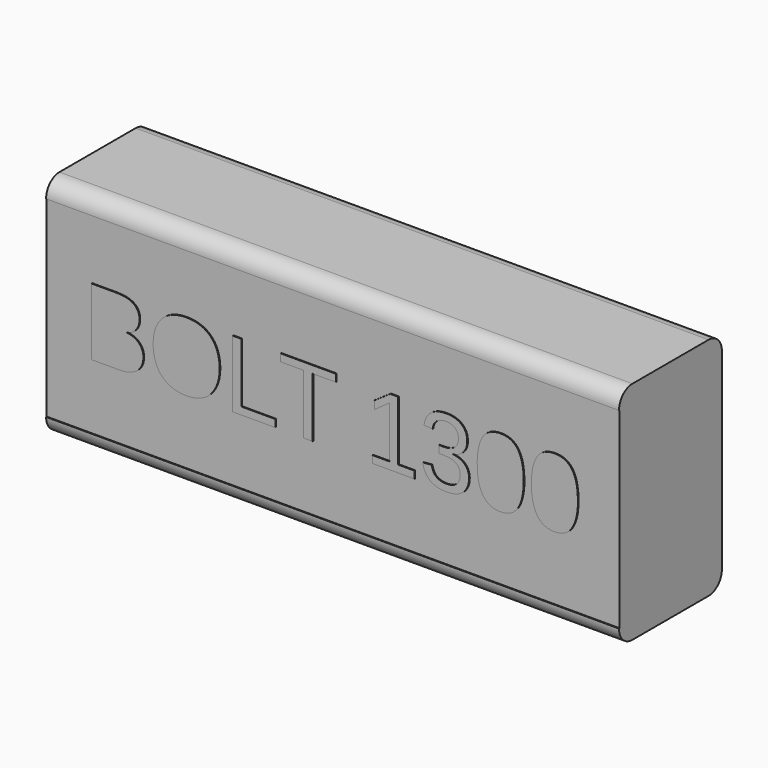
from build123d import *

# Parameters (mm, degrees)
F0_W     = 87.122
F0_H     = 34.29
F1_DEPTH = 9.779
F2_R     = 2.54
F3_W     = 87.122
F3_H     = 29.21
F4_DEPTH = 0.127


with BuildPart() as f1:
    # F0 (on Front) → F1 (new body, symmetric)
    with BuildSketch(Plane.XZ):
        Rectangle(F0_W, F0_H)
    extrude(amount=F1_DEPTH, both=True)

    # F2
    f2_edges = [f1.edges().sort_by_distance(p)[0] for p in [
        (0, 9.779, 17.145),
        (0, 9.779, -17.145),
        (0, -9.779, 17.145),
        (0, -9.779, -17.145),
    ]]
    fillet(f2_edges, radius=F2_R)

    # F3 (on face) → F4 (cut)
    with BuildSketch(Plane.XZ.offset(9.779)):
        Rectangle(F3_W, F3_H)
        with BuildLine():
            add(Edge.make_bspline(
                [(-29.4201796663, -0.1257045448), (-28.7628641118, -0.7945925563), (-28.7628641118, -1.8129687674)],
                knots=[0, 0, 0, 1, 1, 1], degree=2))
            add(Edge.make_bspline(
                [(-28.7628641118, -1.8129687674), (-28.7628641118, -3.1738897042), (-29.7534664263, -3.9295711427)],
                knots=[0, 0, 0, 1, 1, 1], degree=2))
            add(Edge.make_bspline(
                [(-29.7534664263, -3.9295711427), (-30.7440687408, -4.6852525812), (-32.5077111792, -4.6852525812)],
                knots=[0, 0, 0, 1, 1, 1], degree=2))
            Line((-32.5077111792, -4.6852525812), (-36.6460217827, -4.6852525812))
            Line((-36.6460217827, -4.6852525812), (-36.6460217827, 5.5054530046))
            Line((-36.6460217827, 5.5054530046), (-32.9428355603, 5.5054530046))
            add(Edge.make_bspline(
                [(-32.9428355603, 5.5054530046), (-29.3553739074, 5.5054530046), (-29.3553739074, 3.0312617097)],
                knots=[0, 0, 0, 1, 1, 1], degree=2))
            add(Edge.make_bspline(
                [(-29.3553739074, 3.0312617097), (-29.3553739074, 2.128610068), (-29.8610902759, 1.5141126043)],
                knots=[0, 0, 0, 1, 1, 1], degree=2))
            add(Edge.make_bspline(
                [(-29.8610902759, 1.5141126043), (-30.3668066444, 0.8996151405), (-31.2926032, 0.6889964241)],
                knots=[0, 0, 0, 1, 1, 1], degree=2))
            add(Edge.make_bspline(
                [(-31.2926032, 0.6889964241), (-30.0774952208, 0.5431834666), (-29.4201796663, -0.1257045448)],
                knots=[0, 0, 0, 1, 1, 1], degree=2))
        make_face(mode=Mode.SUBTRACT)
        with BuildLine():
            add(Edge.make_bspline(
                [(-17.7713445055, 3.2418804261), (-17.1672622529, 2.0638043091), (-17.1672622529, 0.4575472852)],
                knots=[0, 0, 0, 1, 1, 1], degree=2))
            add(Edge.make_bspline(
                [(-17.1672622529, 0.4575472852), (-17.1672622529, -1.1417662646), (-17.7782879796, -2.3418300498)],
                knots=[0, 0, 0, 1, 1, 1], degree=2))
            add(Edge.make_bspline(
                [(-17.7782879796, -2.3418300498), (-18.3893137063, -3.541893835), (-19.5326724525, -4.1864796868)],
                knots=[0, 0, 0, 1, 1, 1], degree=2))
            add(Edge.make_bspline(
                [(-19.5326724525, -4.1864796868), (-20.6760311986, -4.8310655387), (-22.2313694121, -4.8310655387)],
                knots=[0, 0, 0, 1, 1, 1], degree=2))
            add(Edge.make_bspline(
                [(-22.2313694121, -4.8310655387), (-23.8005945738, -4.8310655387), (-24.9393243372, -4.193423161)],
                knots=[0, 0, 0, 1, 1, 1], degree=2))
            add(Edge.make_bspline(
                [(-24.9393243372, -4.193423161), (-26.0780541006, -3.5557807833), (-26.678664616, -2.3522452611)],
                knots=[0, 0, 0, 1, 1, 1], degree=2))
            add(Edge.make_bspline(
                [(-26.678664616, -2.3522452611), (-27.2792751315, -1.1487097388), (-27.2792751315, 0.4575472852)],
                knots=[0, 0, 0, 1, 1, 1], degree=2))
            add(Edge.make_bspline(
                [(-27.2792751315, 0.4575472852), (-27.2792751315, 2.901650192), (-25.9414991086, 4.2799298141)],
                knots=[0, 0, 0, 1, 1, 1], degree=2))
            add(Edge.make_bspline(
                [(-25.9414991086, 4.2799298141), (-24.6037230858, 5.6582094363), (-22.2151679723, 5.6582094363)],
                knots=[0, 0, 0, 1, 1, 1], degree=2))
            add(Edge.make_bspline(
                [(-22.2151679723, 5.6582094363), (-20.6598297589, 5.6582094363), (-19.5176282585, 5.0390829897)],
                knots=[0, 0, 0, 1, 1, 1], degree=2))
            add(Edge.make_bspline(
                [(-19.5176282585, 5.0390829897), (-18.375426758, 4.4199565431), (-17.7713445055, 3.2418804261)],
                knots=[0, 0, 0, 1, 1, 1], degree=2))
        make_face(mode=Mode.SUBTRACT)
        Polygon((-8.7124252089, -4.6852525812), (-15.2439199087, -4.6852525812), (-15.2439199087, 5.5054530046), (-13.8621685494, 5.5054530046), (-13.8621685494, -3.5557807833), (-8.7124252089, -3.5557807833), align=None, mode=Mode.SUBTRACT)
        Polygon((0.4876780624, 4.3782956981), (-3.0141474092, 4.3782956981), (-3.0141474092, -4.6852525812), (-4.3889552943, -4.6852525812), (-4.3889552943, 4.3782956981), (-7.8884662744, 4.3782956981), (-7.8884662744, 5.5054530046), (0.4876780624, 5.5054530046), align=None, mode=Mode.SUBTRACT)
        Polygon((12.4559130349, -4.6852525812), (6.0702312926, -4.6852525812), (6.0702312926, -3.5789256972), (8.6647761397, -3.5789256972), (8.6647761397, 4.2625711287), (6.3664861904, 2.6192822425), (6.3664861904, 3.8505916615), (8.773557235, 5.5054530046), (9.9747782659, 5.5054530046), (9.9747782659, -3.5789256972), (12.4559130349, -3.5789256972), align=None, mode=Mode.SUBTRACT)
        with BuildLine():
            add(Edge.make_bspline(
                [(20.1284519894, -0.2506870799), (20.7649371214, -0.894115686), (20.7649371214, -1.8708310521)],
                knots=[0, 0, 0, 1, 1, 1], degree=2))
            add(Edge.make_bspline(
                [(20.7649371214, -1.8708310521), (20.7649371214, -3.2826707994), (19.8680717081, -4.0568681691)],
                knots=[0, 0, 0, 1, 1, 1], degree=2))
            add(Edge.make_bspline(
                [(19.8680717081, -4.0568681691), (18.9712062949, -4.8310655387), (17.3070869862, -4.8310655387)],
                knots=[0, 0, 0, 1, 1, 1], degree=2))
            add(Edge.make_bspline(
                [(17.3070869862, -4.8310655387), (15.7610067384, -4.8310655387), (14.8386819198, -4.1320891392)],
                knots=[0, 0, 0, 1, 1, 1], degree=2))
            add(Edge.make_bspline(
                [(14.8386819198, -4.1320891392), (13.9163571013, -3.4331127397), (13.7427702471, -2.0675628202)],
                knots=[0, 0, 0, 1, 1, 1], degree=2))
            Line((13.7427702471, -2.0675628202), (15.0874897442, -1.9448947766))
            add(Edge.make_bspline(
                [(15.0874897442, -1.9448947766), (15.3490272711, -3.7525125514), (17.3070869862, -3.7525125514)],
                knots=[0, 0, 0, 1, 1, 1], degree=2))
            add(Edge.make_bspline(
                [(17.3070869862, -3.7525125514), (18.2907458265, -3.7525125514), (18.8520099884, -3.2676266054)],
                knots=[0, 0, 0, 1, 1, 1], degree=2))
            add(Edge.make_bspline(
                [(18.8520099884, -3.2676266054), (19.4132741502, -2.7827406594), (19.4132741502, -1.8291702071)],
                knots=[0, 0, 0, 1, 1, 1], degree=2))
            add(Edge.make_bspline(
                [(19.4132741502, -1.8291702071), (19.4132741502, -0.9959533071), (18.7733172811, -0.5295832922)],
                knots=[0, 0, 0, 1, 1, 1], degree=2))
            add(Edge.make_bspline(
                [(18.7733172811, -0.5295832922), (18.1333604121, -0.0632132773), (16.925195907, -0.0632132773)],
                knots=[0, 0, 0, 1, 1, 1], degree=2))
            Line((16.925195907, -0.0632132773), (16.1868731539, -0.0632132773))
            Line((16.1868731539, -0.0632132773), (16.1868731539, 1.0639440291))
            Line((16.1868731539, 1.0639440291), (16.895107519, 1.0639440291))
            add(Edge.make_bspline(
                [(16.895107519, 1.0639440291), (17.9667170321, 1.0639440291), (18.5557550906, 1.5314712897)],
                knots=[0, 0, 0, 1, 1, 1], degree=2))
            add(Edge.make_bspline(
                [(18.5557550906, 1.5314712897), (19.1447931491, 1.9989985503), (19.1447931491, 2.8229574847)],
                knots=[0, 0, 0, 1, 1, 1], degree=2))
            add(Edge.make_bspline(
                [(19.1447931491, 2.8229574847), (19.1447931491, 3.6399729451), (18.6645361859, 4.1132864341)],
                knots=[0, 0, 0, 1, 1, 1], degree=2))
            add(Edge.make_bspline(
                [(18.6645361859, 4.1132864341), (18.1842792226, 4.5865999232), (17.2353377531, 4.5865999232)],
                knots=[0, 0, 0, 1, 1, 1], degree=2))
            add(Edge.make_bspline(
                [(17.2353377531, 4.5865999232), (16.3743469564, 4.5865999232), (15.8431711827, 4.1456893136)],
                knots=[0, 0, 0, 1, 1, 1], degree=2))
            add(Edge.make_bspline(
                [(15.8431711827, 4.1456893136), (15.3119954089, 3.7047787039), (15.2240447361, 2.901650192)],
                knots=[0, 0, 0, 1, 1, 1], degree=2))
            Line((15.2240447361, 2.901650192), (13.9163571013, 3.0034878131))
            add(Edge.make_bspline(
                [(13.9163571013, 3.0034878131), (14.0598555674, 4.2556276545), (14.9532492436, 4.9569185454)],
                knots=[0, 0, 0, 1, 1, 1], degree=2))
            add(Edge.make_bspline(
                [(14.9532492436, 4.9569185454), (15.8466429197, 5.6582094363), (17.2492247015, 5.6582094363)],
                knots=[0, 0, 0, 1, 1, 1], degree=2))
            add(Edge.make_bspline(
                [(17.2492247015, 5.6582094363), (18.7837324924, 5.6582094363), (19.6331508322, 4.9453460885)],
                knots=[0, 0, 0, 1, 1, 1], degree=2))
            add(Edge.make_bspline(
                [(19.6331508322, 4.9453460885), (20.4825691719, 4.2324827406), (20.4825691719, 2.9595124767)],
                knots=[0, 0, 0, 1, 1, 1], degree=2))
            add(Edge.make_bspline(
                [(20.4825691719, 2.9595124767), (20.4825691719, 1.9827971105), (19.9363492041, 1.3717713838)],
                knots=[0, 0, 0, 1, 1, 1], degree=2))
            add(Edge.make_bspline(
                [(19.9363492041, 1.3717713838), (19.3901292363, 0.7607456571), (18.3486081113, 0.5431834666)],
                knots=[0, 0, 0, 1, 1, 1], degree=2))
            Line((18.3486081113, 0.5431834666), (18.3486081113, 0.5154095699))
            add(Edge.make_bspline(
                [(18.3486081113, 0.5154095699), (19.4919668574, 0.3927415263), (20.1284519894, -0.2506870799)],
                knots=[0, 0, 0, 1, 1, 1], degree=2))
        make_face(mode=Mode.SUBTRACT)
        with BuildLine():
            add(Edge.make_bspline(
                [(28.2175993939, 4.3343203618), (29.0739612079, 3.0104312872), (29.0739612079, 0.4135719488)],
                knots=[0, 0, 0, 1, 1, 1], degree=2))
            add(Edge.make_bspline(
                [(29.0739612079, 0.4135719488), (29.0739612079, -2.1393120533), (28.1736240576, -3.485188796)],
                knots=[0, 0, 0, 1, 1, 1], degree=2))
            add(Edge.make_bspline(
                [(28.1736240576, -3.485188796), (27.2732869072, -4.8310655387), (25.516587943, -4.8310655387)],
                knots=[0, 0, 0, 1, 1, 1], degree=2))
            add(Edge.make_bspline(
                [(25.516587943, -4.8310655387), (23.7598889787, -4.8310655387), (22.8769105138, -3.4921322701)],
                knots=[0, 0, 0, 1, 1, 1], degree=2))
            add(Edge.make_bspline(
                [(22.8769105138, -3.4921322701), (21.9939320489, -2.1531990016), (21.9939320489, 0.4135719488)],
                knots=[0, 0, 0, 1, 1, 1], degree=2))
            add(Edge.make_bspline(
                [(21.9939320489, 0.4135719488), (21.9939320489, 3.0405196753), (22.8514511086, 4.3493645558)],
                knots=[0, 0, 0, 1, 1, 1], degree=2))
            add(Edge.make_bspline(
                [(22.8514511086, 4.3493645558), (23.7089701682, 5.6582094363), (25.5605632794, 5.6582094363)],
                knots=[0, 0, 0, 1, 1, 1], degree=2))
            add(Edge.make_bspline(
                [(25.5605632794, 5.6582094363), (27.36123758, 5.6582094363), (28.2175993939, 4.3343203618)],
                knots=[0, 0, 0, 1, 1, 1], degree=2))
        make_face(mode=Mode.SUBTRACT)
        with BuildLine():
            add(Edge.make_bspline(
                [(36.4548742474, 4.3343203618), (37.3112360613, 3.0104312872), (37.3112360613, 0.4135719488)],
                knots=[0, 0, 0, 1, 1, 1], degree=2))
            add(Edge.make_bspline(
                [(37.3112360613, 0.4135719488), (37.3112360613, -2.1393120533), (36.410898911, -3.485188796)],
                knots=[0, 0, 0, 1, 1, 1], degree=2))
            add(Edge.make_bspline(
                [(36.410898911, -3.485188796), (35.5105617607, -4.8310655387), (33.7538627964, -4.8310655387)],
                knots=[0, 0, 0, 1, 1, 1], degree=2))
            add(Edge.make_bspline(
                [(33.7538627964, -4.8310655387), (31.9971638322, -4.8310655387), (31.1141853673, -3.4921322701)],
                knots=[0, 0, 0, 1, 1, 1], degree=2))
            add(Edge.make_bspline(
                [(31.1141853673, -3.4921322701), (30.2312069024, -2.1531990016), (30.2312069024, 0.4135719488)],
                knots=[0, 0, 0, 1, 1, 1], degree=2))
            add(Edge.make_bspline(
                [(30.2312069024, 0.4135719488), (30.2312069024, 3.0405196753), (31.088725962, 4.3493645558)],
                knots=[0, 0, 0, 1, 1, 1], degree=2))
            add(Edge.make_bspline(
                [(31.088725962, 4.3493645558), (31.9462450216, 5.6582094363), (33.7978381328, 5.6582094363)],
                knots=[0, 0, 0, 1, 1, 1], degree=2))
            add(Edge.make_bspline(
                [(33.7978381328, 5.6582094363), (35.5985124335, 5.6582094363), (36.4548742474, 4.3343203618)],
                knots=[0, 0, 0, 1, 1, 1], degree=2))
        make_face(mode=Mode.SUBTRACT)
    extrude(amount=-F4_DEPTH, mode=Mode.SUBTRACT)


with BuildPart() as f5_1:
    # F5: copy of F1
    add(f1.part)


solid = Compound([f1.part, f5_1.part])
